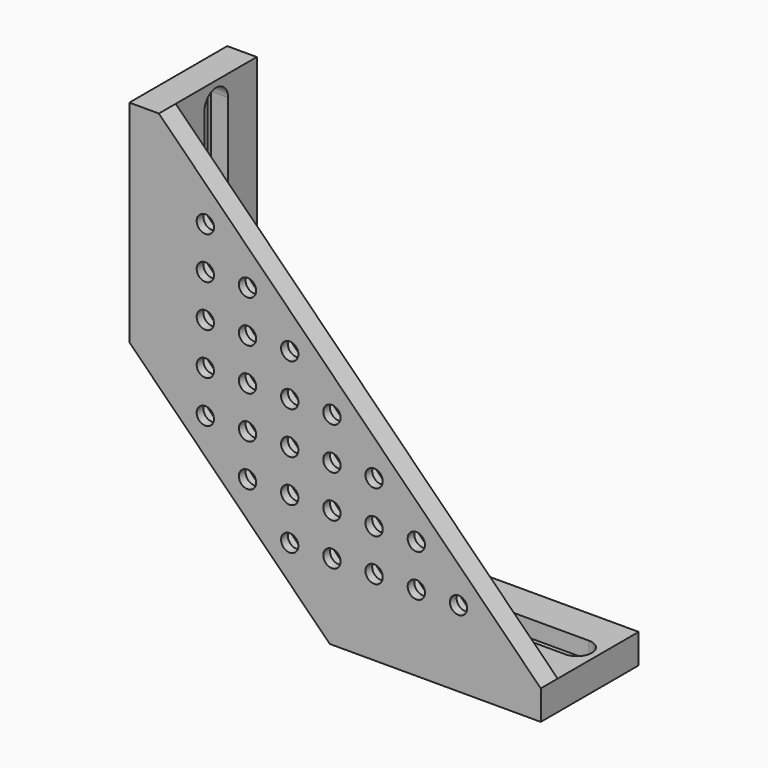
from build123d import *

# Parameters (mm, degrees)
F1_DEPTH  = 7
F2_DEPTH  = 3
F4_ANGLE  = 90
F8_ANGLE  = 180
F12_R     = 2.05
F13_DEPTH = 5
F14_DEPTH = 3


# Not quite as in the source:
# - a feature names something its author has since deleted; it is built from what else it names


with BuildPart() as f1:
    # F0 (on Top) → F1 (new body)
    with BuildSketch(Plane.XY):
        Polygon((29, 12), (-21, 12), (-21, -12), (0, -12), (29, -12), align=None)
        with BuildLine():
            ThreePointArc((-16, -11.5), (-19.5, -8), (-16, -4.5))
            Line((-16, -4.5), (0, -4.5))
            Line((0, -4.5), (24, -4.5))
            ThreePointArc((24, -4.5), (27.5, -8), (24, -11.5))
            Line((24, -11.5), (0, -11.5))
            Line((0, -11.5), (-16, -11.5))
        make_face(mode=Mode.SUBTRACT)
        with BuildLine():
            Line((24, -3.5), (-16, -3.5))
            ThreePointArc((-16, -3.5), (-19.5, 0), (-16, 3.5))
            Line((-16, 3.5), (24, 3.5))
            ThreePointArc((24, 3.5), (27.5, 0), (24, -3.5))
        make_face(mode=Mode.SUBTRACT)
        with BuildLine():
            Line((0, 4.5), (-16, 4.5))
            ThreePointArc((-16, 4.5), (-19.5, 8), (-16, 11.5))
            Line((-16, 11.5), (0, 11.5))
            Line((0, 11.5), (24, 11.5))
            ThreePointArc((24, 11.5), (27.5, 8), (24, 4.5))
            Line((24, 4.5), (0, 4.5))
        make_face(mode=Mode.SUBTRACT)
        with BuildLine():
            Line((0, -4.5), (-16, -4.5))
            ThreePointArc((-16, -4.5), (-19.5, -8), (-16, -11.5))
            Line((-16, -11.5), (0, -11.5))
            Line((0, -11.5), (24, -11.5))
            ThreePointArc((24, -11.5), (27.5, -8), (24, -4.5))
            Line((24, -4.5), (0, -4.5))
        make_face()
        with BuildLine():
            ThreePointArc((-16, -10.05), (-18.05, -8), (-16, -5.95))
            Line((-16, -5.95), (0, -5.95))
            Line((0, -5.95), (24, -5.95))
            ThreePointArc((24, -5.95), (26.05, -8), (24, -10.05))
            Line((24, -10.05), (0, -10.05))
            Line((0, -10.05), (-16, -10.05))
        make_face(mode=Mode.SUBTRACT)
        with BuildLine():
            ThreePointArc((-16, 11.5), (-19.5, 8), (-16, 4.5))
            Line((-16, 4.5), (0, 4.5))
            Line((0, 4.5), (24, 4.5))
            ThreePointArc((24, 4.5), (27.5, 8), (24, 11.5))
            Line((24, 11.5), (0, 11.5))
            Line((0, 11.5), (-16, 11.5))
        make_face()
        with BuildLine():
            Line((24, 5.95), (0, 5.95))
            Line((0, 5.95), (-16, 5.95))
            ThreePointArc((-16, 5.95), (-18.05, 8), (-16, 10.05))
            Line((-16, 10.05), (0, 10.05))
            Line((0, 10.05), (24, 10.05))
            ThreePointArc((24, 10.05), (26.05, 8), (24, 5.95))
        make_face(mode=Mode.SUBTRACT)
        with BuildLine():
            Line((0, -5.95), (-16, -5.95))
            ThreePointArc((-16, -5.95), (-18.05, -8), (-16, -10.05))
            Line((-16, -10.05), (0, -10.05))
            Line((0, -10.05), (24, -10.05))
            ThreePointArc((24, -10.05), (26.05, -8), (24, -5.95))
            Line((24, -5.95), (0, -5.95))
        make_face()
        with BuildLine():
            Line((-16, 5.95), (0, 5.95))
            Line((0, 5.95), (24, 5.95))
            ThreePointArc((24, 5.95), (26.05, 8), (24, 10.05))
            Line((24, 10.05), (0, 10.05))
            Line((0, 10.05), (-16, 10.05))
            ThreePointArc((-16, 10.05), (-18.05, 8), (-16, 5.95))
        make_face()
    extrude(amount=F1_DEPTH)

    # F0 (on Top) → F2 (join)
    with BuildSketch(Plane.XY):
        with BuildLine():
            ThreePointArc((-16, 3.5), (-19.5, 0), (-16, -3.5))
            Line((-16, -3.5), (24, -3.5))
            ThreePointArc((24, -3.5), (27.5, 0), (24, 3.5))
            Line((24, 3.5), (-16, 3.5))
        make_face()
        with BuildLine():
            Line((0, -2.45), (-16, -2.45))
            ThreePointArc((-16, -2.45), (-18.45, 0), (-16, 2.45))
            Line((-16, 2.45), (0, 2.45))
            Line((0, 2.45), (24, 2.45))
            ThreePointArc((24, 2.45), (26.45, 0), (24, -2.45))
            Line((24, -2.45), (0, -2.45))
        make_face(mode=Mode.SUBTRACT)
    extrude(amount=F2_DEPTH)


with BuildPart() as f4_1:
    # F4: copy of F1
    add(f1.part.rotate(Axis((-21, 0, 3.5), (0, -1, 0)), F4_ANGLE))


with BuildPart() as f4_1_1:
    # F8: moved
    add(f4_1.part.rotate(Axis((-21, 0, 28.5), (0, 0, 1)), F8_ANGLE))


with BuildPart() as f4_1_2:
    # F9: moved
    add(f4_1_1.part.moved(Location((0, 0, 44))))


with BuildPart() as f4_1_3:
    # F10: moved
    add(f4_1_2.part.moved(Location((-44, 0, 0))))


with BuildPart() as f1_1:
    add(f1.part)

    add(f4_1_3.part)  # F13 merges F4_1
    # F12 (on 3pt) → F13 (join)
    with BuildSketch(Plane.XZ.offset(12)):
        Polygon((-68.5, 47.5), (-21, 0), (29, 0), (29, 7), (-61.5, 97.5), (-68.5, 97.5), align=None)
        Polygon((-34.3563439923, 16.9720831325), (-33.3210678119, 20.8357864376), (-29.4573645067, 21.871062618), (-26.628937382, 19.0426354933), (-27.6642135624, 15.1789321881), (-31.5279168675, 14.1436560077), align=None, mode=Mode.SUBTRACT)
        Polygon((-24.3563439923, 16.9720831325), (-23.3210678119, 20.8357864376), (-19.4573645067, 21.871062618), (-16.628937382, 19.0426354933), (-17.6642135624, 15.1789321881), (-21.5279168675, 14.1436560077), align=None, mode=Mode.SUBTRACT)
        Polygon((-54.3563439923, 36.9720831325), (-53.3210678119, 40.8357864376), (-49.4573645067, 41.871062618), (-46.628937382, 39.0426354933), (-47.6642135624, 35.1789321881), (-51.5279168675, 34.1436560077), align=None, mode=Mode.SUBTRACT)
        Polygon((-54.3563439923, 46.9720831325), (-53.3210678119, 50.8357864376), (-49.4573645067, 51.871062618), (-46.628937382, 49.0426354933), (-47.6642135624, 45.1789321881), (-51.5279168675, 44.1436560077), align=None, mode=Mode.SUBTRACT)
        Polygon((-44.3563439923, 26.9720831325), (-43.3210678119, 30.8357864376), (-39.4573645067, 31.871062618), (-36.628937382, 29.0426354933), (-37.6642135624, 25.1789321881), (-41.5279168675, 24.1436560077), align=None, mode=Mode.SUBTRACT)
        Polygon((-34.3563439923, 26.9720831325), (-33.3210678119, 30.8357864376), (-29.4573645067, 31.871062618), (-26.628937382, 29.0426354933), (-27.6642135624, 25.1789321881), (-31.5279168675, 24.1436560077), align=None, mode=Mode.SUBTRACT)
        Polygon((-24.3563439923, 26.9720831325), (-23.3210678119, 30.8357864376), (-19.4573645067, 31.871062618), (-16.628937382, 29.0426354933), (-17.6642135624, 25.1789321881), (-21.5279168675, 24.1436560077), align=None, mode=Mode.SUBTRACT)
        Polygon((-44.3563439923, 36.9720831325), (-43.3210678119, 40.8357864376), (-39.4573645067, 41.871062618), (-36.628937382, 39.0426354933), (-37.6642135624, 35.1789321881), (-41.5279168675, 34.1436560077), align=None, mode=Mode.SUBTRACT)
        Polygon((-44.3563439923, 46.9720831325), (-43.3210678119, 50.8357864376), (-39.4573645067, 51.871062618), (-36.628937382, 49.0426354933), (-37.6642135624, 45.1789321881), (-41.5279168675, 44.1436560077), align=None, mode=Mode.SUBTRACT)
        Polygon((-34.3563439923, 36.9720831325), (-33.3210678119, 40.8357864376), (-29.4573645067, 41.871062618), (-26.628937382, 39.0426354933), (-27.6642135624, 35.1789321881), (-31.5279168675, 34.1436560077), align=None, mode=Mode.SUBTRACT)
        Polygon((-24.3563439923, 36.9720831325), (-23.3210678119, 40.8357864376), (-19.4573645067, 41.871062618), (-16.628937382, 39.0426354933), (-17.6642135624, 35.1789321881), (-21.5279168675, 34.1436560077), align=None, mode=Mode.SUBTRACT)
        Polygon((-34.3563439923, 46.9720831325), (-33.3210678119, 50.8357864376), (-29.4573645067, 51.871062618), (-26.628937382, 49.0426354933), (-27.6642135624, 45.1789321881), (-31.5279168675, 44.1436560077), align=None, mode=Mode.SUBTRACT)
        Polygon((-24.3563439923, 46.9720831325), (-23.3210678119, 50.8357864376), (-19.4573645067, 51.871062618), (-16.628937382, 49.0426354933), (-17.6642135624, 45.1789321881), (-21.5279168675, 44.1436560077), align=None, mode=Mode.SUBTRACT)
        Polygon((-14.3563439923, 16.9720831325), (-13.3210678119, 20.8357864376), (-9.4573645067, 21.871062618), (-6.628937382, 19.0426354933), (-7.6642135624, 15.1789321881), (-11.5279168675, 14.1436560077), align=None, mode=Mode.SUBTRACT)
        Polygon((-4.3563439923, 16.9720831325), (-3.3210678119, 20.8357864376), (0.5426354933, 21.871062618), (3.371062618, 19.0426354933), (2.3357864376, 15.1789321881), (-1.5279168675, 14.1436560077), align=None, mode=Mode.SUBTRACT)
        Polygon((8.4720831325, 14.1436560077), (5.6436560077, 16.9720831325), (6.6789321881, 20.8357864376), (10.5426354933, 21.871062618), (13.371062618, 19.0426354933), (12.3357864376, 15.1789321881), align=None, mode=Mode.SUBTRACT)
        Polygon((-14.3563439923, 26.9720831325), (-13.3210678119, 30.8357864376), (-9.4573645067, 31.871062618), (-6.628937382, 29.0426354933), (-7.6642135624, 25.1789321881), (-11.5279168675, 24.1436560077), align=None, mode=Mode.SUBTRACT)
        Polygon((-4.3563439923, 26.9720831325), (-3.3210678119, 30.8357864376), (0.5426354933, 31.871062618), (3.371062618, 29.0426354933), (2.3357864376, 25.1789321881), (-1.5279168675, 24.1436560077), align=None, mode=Mode.SUBTRACT)
        Polygon((-14.3563439923, 36.9720831325), (-13.3210678119, 40.8357864376), (-9.4573645067, 41.871062618), (-6.628937382, 39.0426354933), (-7.6642135624, 35.1789321881), (-11.5279168675, 34.1436560077), align=None, mode=Mode.SUBTRACT)
        Polygon((-54.3563439923, 56.9720831325), (-53.3210678119, 60.8357864376), (-49.4573645067, 61.871062618), (-46.628937382, 59.0426354933), (-47.6642135624, 55.1789321881), (-51.5279168675, 54.1436560077), align=None, mode=Mode.SUBTRACT)
        Polygon((-54.3563439923, 66.9720831325), (-53.3210678119, 70.8357864376), (-49.4573645067, 71.871062618), (-46.628937382, 69.0426354933), (-47.6642135624, 65.1789321881), (-51.5279168675, 64.1436560077), align=None, mode=Mode.SUBTRACT)
        Polygon((-44.3563439923, 56.9720831325), (-43.3210678119, 60.8357864376), (-39.4573645067, 61.871062618), (-36.628937382, 59.0426354933), (-37.6642135624, 55.1789321881), (-41.5279168675, 54.1436560077), align=None, mode=Mode.SUBTRACT)
        Polygon((-34.3563439923, 56.9720831325), (-33.3210678119, 60.8357864376), (-29.4573645067, 61.871062618), (-26.628937382, 59.0426354933), (-27.6642135624, 55.1789321881), (-31.5279168675, 54.1436560077), align=None, mode=Mode.SUBTRACT)
        Polygon((-41.5279168675, 64.1436560077), (-44.3563439923, 66.9720831325), (-43.3210678119, 70.8357864376), (-39.4573645067, 71.871062618), (-36.628937382, 69.0426354933), (-37.6642135624, 65.1789321881), align=None, mode=Mode.SUBTRACT)
        Polygon((-51.5279168675, 74.1436560077), (-54.3563439923, 76.9720831325), (-53.3210678119, 80.8357864376), (-49.4573645067, 81.871062618), (-46.628937382, 79.0426354933), (-47.6642135624, 75.1789321881), align=None, mode=Mode.SUBTRACT)
        Polygon((-19.4573645067, 51.871062618), (-23.3210678119, 50.8357864376), (-24.3563439923, 46.9720831325), (-21.5279168675, 44.1436560077), (-17.6642135624, 45.1789321881), (-16.628937382, 49.0426354933), align=None)
        with Locations((-20.4926406871, 48.0073593129)):
            Circle(F12_R, mode=Mode.SUBTRACT)
        Polygon((-29.4573645067, 61.871062618), (-33.3210678119, 60.8357864376), (-34.3563439923, 56.9720831325), (-31.5279168675, 54.1436560077), (-27.6642135624, 55.1789321881), (-26.628937382, 59.0426354933), align=None)
        with Locations((-30.4926406871, 58.0073593129)):
            Circle(F12_R, mode=Mode.SUBTRACT)
        Polygon((-29.4573645067, 51.871062618), (-33.3210678119, 50.8357864376), (-34.3563439923, 46.9720831325), (-31.5279168675, 44.1436560077), (-27.6642135624, 45.1789321881), (-26.628937382, 49.0426354933), align=None)
        with Locations((-30.4926406871, 48.0073593129)):
            Circle(F12_R, mode=Mode.SUBTRACT)
        Polygon((-29.4573645067, 41.871062618), (-33.3210678119, 40.8357864376), (-34.3563439923, 36.9720831325), (-31.5279168675, 34.1436560077), (-27.6642135624, 35.1789321881), (-26.628937382, 39.0426354933), align=None)
        with Locations((-30.4926406871, 38.0073593129)):
            Circle(F12_R, mode=Mode.SUBTRACT)
        Polygon((-19.4573645067, 41.871062618), (-23.3210678119, 40.8357864376), (-24.3563439923, 36.9720831325), (-21.5279168675, 34.1436560077), (-17.6642135624, 35.1789321881), (-16.628937382, 39.0426354933), align=None)
        with Locations((-20.4926406871, 38.0073593129)):
            Circle(F12_R, mode=Mode.SUBTRACT)
        Polygon((-9.4573645067, 41.871062618), (-13.3210678119, 40.8357864376), (-14.3563439923, 36.9720831325), (-11.5279168675, 34.1436560077), (-7.6642135624, 35.1789321881), (-6.628937382, 39.0426354933), align=None)
        with Locations((-10.4926406871, 38.0073593129)):
            Circle(F12_R, mode=Mode.SUBTRACT)
        Polygon((-43.3210678119, 70.8357864376), (-44.3563439923, 66.9720831325), (-41.5279168675, 64.1436560077), (-37.6642135624, 65.1789321881), (-36.628937382, 69.0426354933), (-39.4573645067, 71.871062618), align=None)
        with Locations((-40.4926406871, 68.0073593129)):
            Circle(F12_R, mode=Mode.SUBTRACT)
        Polygon((-39.4573645067, 61.871062618), (-43.3210678119, 60.8357864376), (-44.3563439923, 56.9720831325), (-41.5279168675, 54.1436560077), (-37.6642135624, 55.1789321881), (-36.628937382, 59.0426354933), align=None)
        with Locations((-40.4926406871, 58.0073593129)):
            Circle(F12_R, mode=Mode.SUBTRACT)
        Polygon((-39.4573645067, 51.871062618), (-43.3210678119, 50.8357864376), (-44.3563439923, 46.9720831325), (-41.5279168675, 44.1436560077), (-37.6642135624, 45.1789321881), (-36.628937382, 49.0426354933), align=None)
        with Locations((-40.4926406871, 48.0073593129)):
            Circle(F12_R, mode=Mode.SUBTRACT)
        Polygon((-39.4573645067, 41.871062618), (-43.3210678119, 40.8357864376), (-44.3563439923, 36.9720831325), (-41.5279168675, 34.1436560077), (-37.6642135624, 35.1789321881), (-36.628937382, 39.0426354933), align=None)
        with Locations((-40.4926406871, 38.0073593129)):
            Circle(F12_R, mode=Mode.SUBTRACT)
        Polygon((-39.4573645067, 31.871062618), (-43.3210678119, 30.8357864376), (-44.3563439923, 26.9720831325), (-41.5279168675, 24.1436560077), (-37.6642135624, 25.1789321881), (-36.628937382, 29.0426354933), align=None)
        with Locations((-40.4926406871, 28.0073593129)):
            Circle(F12_R, mode=Mode.SUBTRACT)
        Polygon((-29.4573645067, 31.871062618), (-33.3210678119, 30.8357864376), (-34.3563439923, 26.9720831325), (-31.5279168675, 24.1436560077), (-27.6642135624, 25.1789321881), (-26.628937382, 29.0426354933), align=None)
        with Locations((-30.4926406871, 28.0073593129)):
            Circle(F12_R, mode=Mode.SUBTRACT)
        Polygon((-19.4573645067, 31.871062618), (-23.3210678119, 30.8357864376), (-24.3563439923, 26.9720831325), (-21.5279168675, 24.1436560077), (-17.6642135624, 25.1789321881), (-16.628937382, 29.0426354933), align=None)
        with Locations((-20.4926406871, 28.0073593129)):
            Circle(F12_R, mode=Mode.SUBTRACT)
        Polygon((-9.4573645067, 31.871062618), (-13.3210678119, 30.8357864376), (-14.3563439923, 26.9720831325), (-11.5279168675, 24.1436560077), (-7.6642135624, 25.1789321881), (-6.628937382, 29.0426354933), align=None)
        with Locations((-10.4926406871, 28.0073593129)):
            Circle(F12_R, mode=Mode.SUBTRACT)
        Polygon((0.5426354933, 31.871062618), (-3.3210678119, 30.8357864376), (-4.3563439923, 26.9720831325), (-1.5279168675, 24.1436560077), (2.3357864376, 25.1789321881), (3.371062618, 29.0426354933), align=None)
        with Locations((-0.4926406871, 28.0073593129)):
            Circle(F12_R, mode=Mode.SUBTRACT)
        Polygon((-49.4573645067, 61.871062618), (-53.3210678119, 60.8357864376), (-54.3563439923, 56.9720831325), (-51.5279168675, 54.1436560077), (-47.6642135624, 55.1789321881), (-46.628937382, 59.0426354933), align=None)
        with Locations((-50.4926406871, 58.0073593129)):
            Circle(F12_R, mode=Mode.SUBTRACT)
        Polygon((-49.4573645067, 71.871062618), (-53.3210678119, 70.8357864376), (-54.3563439923, 66.9720831325), (-51.5279168675, 64.1436560077), (-47.6642135624, 65.1789321881), (-46.628937382, 69.0426354933), align=None)
        with Locations((-50.4926406871, 68.0073593129)):
            Circle(F12_R, mode=Mode.SUBTRACT)
        Polygon((-53.3210678119, 80.8357864376), (-54.3563439923, 76.9720831325), (-51.5279168675, 74.1436560077), (-47.6642135624, 75.1789321881), (-46.628937382, 79.0426354933), (-49.4573645067, 81.871062618), align=None)
        with Locations((-50.4926406871, 78.0073593129)):
            Circle(F12_R, mode=Mode.SUBTRACT)
        Polygon((-49.4573645067, 51.871062618), (-53.3210678119, 50.8357864376), (-54.3563439923, 46.9720831325), (-51.5279168675, 44.1436560077), (-47.6642135624, 45.1789321881), (-46.628937382, 49.0426354933), align=None)
        with Locations((-50.4926406871, 48.0073593129)):
            Circle(F12_R, mode=Mode.SUBTRACT)
        Polygon((-49.4573645067, 41.871062618), (-53.3210678119, 40.8357864376), (-54.3563439923, 36.9720831325), (-51.5279168675, 34.1436560077), (-47.6642135624, 35.1789321881), (-46.628937382, 39.0426354933), align=None)
        with Locations((-50.4926406871, 38.0073593129)):
            Circle(F12_R, mode=Mode.SUBTRACT)
        Polygon((-29.4573645067, 21.871062618), (-33.3210678119, 20.8357864376), (-34.3563439923, 16.9720831325), (-31.5279168675, 14.1436560077), (-27.6642135624, 15.1789321881), (-26.628937382, 19.0426354933), align=None)
        with Locations((-30.4926406871, 18.0073593129)):
            Circle(F12_R, mode=Mode.SUBTRACT)
        Polygon((-19.4573645067, 21.871062618), (-23.3210678119, 20.8357864376), (-24.3563439923, 16.9720831325), (-21.5279168675, 14.1436560077), (-17.6642135624, 15.1789321881), (-16.628937382, 19.0426354933), align=None)
        with Locations((-20.4926406871, 18.0073593129)):
            Circle(F12_R, mode=Mode.SUBTRACT)
        Polygon((-9.4573645067, 21.871062618), (-13.3210678119, 20.8357864376), (-14.3563439923, 16.9720831325), (-11.5279168675, 14.1436560077), (-7.6642135624, 15.1789321881), (-6.628937382, 19.0426354933), align=None)
        with Locations((-10.4926406871, 18.0073593129)):
            Circle(F12_R, mode=Mode.SUBTRACT)
        Polygon((0.5426354933, 21.871062618), (-3.3210678119, 20.8357864376), (-4.3563439923, 16.9720831325), (-1.5279168675, 14.1436560077), (2.3357864376, 15.1789321881), (3.371062618, 19.0426354933), align=None)
        with Locations((-0.4926406871, 18.0073593129)):
            Circle(F12_R, mode=Mode.SUBTRACT)
        Polygon((6.6789321881, 20.8357864376), (5.6436560077, 16.9720831325), (8.4720831325, 14.1436560077), (12.3357864376, 15.1789321881), (13.371062618, 19.0426354933), (10.5426354933, 21.871062618), align=None)
        with Locations((9.5073593129, 18.0073593129)):
            Circle(F12_R, mode=Mode.SUBTRACT)
    extrude(amount=F13_DEPTH)

    # F12 (on 3pt) → F14 (cut)
    with BuildSketch(Plane.XZ.offset(12)):
        Polygon((-19.4573645067, 51.871062618), (-23.3210678119, 50.8357864376), (-24.3563439923, 46.9720831325), (-21.5279168675, 44.1436560077), (-17.6642135624, 45.1789321881), (-16.628937382, 49.0426354933), align=None)
        with Locations((-20.4926406871, 48.0073593129)):
            Circle(F12_R, mode=Mode.SUBTRACT)
        Polygon((-9.4573645067, 41.871062618), (-13.3210678119, 40.8357864376), (-14.3563439923, 36.9720831325), (-11.5279168675, 34.1436560077), (-7.6642135624, 35.1789321881), (-6.628937382, 39.0426354933), align=None)
        with Locations((-10.4926406871, 38.0073593129)):
            Circle(F12_R, mode=Mode.SUBTRACT)
        Polygon((-19.4573645067, 41.871062618), (-23.3210678119, 40.8357864376), (-24.3563439923, 36.9720831325), (-21.5279168675, 34.1436560077), (-17.6642135624, 35.1789321881), (-16.628937382, 39.0426354933), align=None)
        with Locations((-20.4926406871, 38.0073593129)):
            Circle(F12_R, mode=Mode.SUBTRACT)
        Polygon((-29.4573645067, 41.871062618), (-33.3210678119, 40.8357864376), (-34.3563439923, 36.9720831325), (-31.5279168675, 34.1436560077), (-27.6642135624, 35.1789321881), (-26.628937382, 39.0426354933), align=None)
        with Locations((-30.4926406871, 38.0073593129)):
            Circle(F12_R, mode=Mode.SUBTRACT)
        Polygon((-29.4573645067, 51.871062618), (-33.3210678119, 50.8357864376), (-34.3563439923, 46.9720831325), (-31.5279168675, 44.1436560077), (-27.6642135624, 45.1789321881), (-26.628937382, 49.0426354933), align=None)
        with Locations((-30.4926406871, 48.0073593129)):
            Circle(F12_R, mode=Mode.SUBTRACT)
        Polygon((-29.4573645067, 61.871062618), (-33.3210678119, 60.8357864376), (-34.3563439923, 56.9720831325), (-31.5279168675, 54.1436560077), (-27.6642135624, 55.1789321881), (-26.628937382, 59.0426354933), align=None)
        with Locations((-30.4926406871, 58.0073593129)):
            Circle(F12_R, mode=Mode.SUBTRACT)
        Polygon((0.5426354933, 31.871062618), (-3.3210678119, 30.8357864376), (-4.3563439923, 26.9720831325), (-1.5279168675, 24.1436560077), (2.3357864376, 25.1789321881), (3.371062618, 29.0426354933), align=None)
        with Locations((-0.4926406871, 28.0073593129)):
            Circle(F12_R, mode=Mode.SUBTRACT)
        Polygon((-9.4573645067, 31.871062618), (-13.3210678119, 30.8357864376), (-14.3563439923, 26.9720831325), (-11.5279168675, 24.1436560077), (-7.6642135624, 25.1789321881), (-6.628937382, 29.0426354933), align=None)
        with Locations((-10.4926406871, 28.0073593129)):
            Circle(F12_R, mode=Mode.SUBTRACT)
        Polygon((-19.4573645067, 31.871062618), (-23.3210678119, 30.8357864376), (-24.3563439923, 26.9720831325), (-21.5279168675, 24.1436560077), (-17.6642135624, 25.1789321881), (-16.628937382, 29.0426354933), align=None)
        with Locations((-20.4926406871, 28.0073593129)):
            Circle(F12_R, mode=Mode.SUBTRACT)
        Polygon((-29.4573645067, 31.871062618), (-33.3210678119, 30.8357864376), (-34.3563439923, 26.9720831325), (-31.5279168675, 24.1436560077), (-27.6642135624, 25.1789321881), (-26.628937382, 29.0426354933), align=None)
        with Locations((-30.4926406871, 28.0073593129)):
            Circle(F12_R, mode=Mode.SUBTRACT)
        Polygon((-39.4573645067, 31.871062618), (-43.3210678119, 30.8357864376), (-44.3563439923, 26.9720831325), (-41.5279168675, 24.1436560077), (-37.6642135624, 25.1789321881), (-36.628937382, 29.0426354933), align=None)
        with Locations((-40.4926406871, 28.0073593129)):
            Circle(F12_R, mode=Mode.SUBTRACT)
        Polygon((-39.4573645067, 41.871062618), (-43.3210678119, 40.8357864376), (-44.3563439923, 36.9720831325), (-41.5279168675, 34.1436560077), (-37.6642135624, 35.1789321881), (-36.628937382, 39.0426354933), align=None)
        with Locations((-40.4926406871, 38.0073593129)):
            Circle(F12_R, mode=Mode.SUBTRACT)
        Polygon((-39.4573645067, 51.871062618), (-43.3210678119, 50.8357864376), (-44.3563439923, 46.9720831325), (-41.5279168675, 44.1436560077), (-37.6642135624, 45.1789321881), (-36.628937382, 49.0426354933), align=None)
        with Locations((-40.4926406871, 48.0073593129)):
            Circle(F12_R, mode=Mode.SUBTRACT)
        Polygon((-39.4573645067, 61.871062618), (-43.3210678119, 60.8357864376), (-44.3563439923, 56.9720831325), (-41.5279168675, 54.1436560077), (-37.6642135624, 55.1789321881), (-36.628937382, 59.0426354933), align=None)
        with Locations((-40.4926406871, 58.0073593129)):
            Circle(F12_R, mode=Mode.SUBTRACT)
        Polygon((-43.3210678119, 70.8357864376), (-44.3563439923, 66.9720831325), (-41.5279168675, 64.1436560077), (-37.6642135624, 65.1789321881), (-36.628937382, 69.0426354933), (-39.4573645067, 71.871062618), align=None)
        with Locations((-40.4926406871, 68.0073593129)):
            Circle(F12_R, mode=Mode.SUBTRACT)
        Polygon((-53.3210678119, 80.8357864376), (-54.3563439923, 76.9720831325), (-51.5279168675, 74.1436560077), (-47.6642135624, 75.1789321881), (-46.628937382, 79.0426354933), (-49.4573645067, 81.871062618), align=None)
        with Locations((-50.4926406871, 78.0073593129)):
            Circle(F12_R, mode=Mode.SUBTRACT)
        Polygon((-49.4573645067, 71.871062618), (-53.3210678119, 70.8357864376), (-54.3563439923, 66.9720831325), (-51.5279168675, 64.1436560077), (-47.6642135624, 65.1789321881), (-46.628937382, 69.0426354933), align=None)
        with Locations((-50.4926406871, 68.0073593129)):
            Circle(F12_R, mode=Mode.SUBTRACT)
        Polygon((-49.4573645067, 61.871062618), (-53.3210678119, 60.8357864376), (-54.3563439923, 56.9720831325), (-51.5279168675, 54.1436560077), (-47.6642135624, 55.1789321881), (-46.628937382, 59.0426354933), align=None)
        with Locations((-50.4926406871, 58.0073593129)):
            Circle(F12_R, mode=Mode.SUBTRACT)
        Polygon((-49.4573645067, 51.871062618), (-53.3210678119, 50.8357864376), (-54.3563439923, 46.9720831325), (-51.5279168675, 44.1436560077), (-47.6642135624, 45.1789321881), (-46.628937382, 49.0426354933), align=None)
        with Locations((-50.4926406871, 48.0073593129)):
            Circle(F12_R, mode=Mode.SUBTRACT)
        Polygon((-49.4573645067, 41.871062618), (-53.3210678119, 40.8357864376), (-54.3563439923, 36.9720831325), (-51.5279168675, 34.1436560077), (-47.6642135624, 35.1789321881), (-46.628937382, 39.0426354933), align=None)
        with Locations((-50.4926406871, 38.0073593129)):
            Circle(F12_R, mode=Mode.SUBTRACT)
        Polygon((-29.4573645067, 21.871062618), (-33.3210678119, 20.8357864376), (-34.3563439923, 16.9720831325), (-31.5279168675, 14.1436560077), (-27.6642135624, 15.1789321881), (-26.628937382, 19.0426354933), align=None)
        with Locations((-30.4926406871, 18.0073593129)):
            Circle(F12_R, mode=Mode.SUBTRACT)
        Polygon((-19.4573645067, 21.871062618), (-23.3210678119, 20.8357864376), (-24.3563439923, 16.9720831325), (-21.5279168675, 14.1436560077), (-17.6642135624, 15.1789321881), (-16.628937382, 19.0426354933), align=None)
        with Locations((-20.4926406871, 18.0073593129)):
            Circle(F12_R, mode=Mode.SUBTRACT)
        Polygon((-9.4573645067, 21.871062618), (-13.3210678119, 20.8357864376), (-14.3563439923, 16.9720831325), (-11.5279168675, 14.1436560077), (-7.6642135624, 15.1789321881), (-6.628937382, 19.0426354933), align=None)
        with Locations((-10.4926406871, 18.0073593129)):
            Circle(F12_R, mode=Mode.SUBTRACT)
        Polygon((0.5426354933, 21.871062618), (-3.3210678119, 20.8357864376), (-4.3563439923, 16.9720831325), (-1.5279168675, 14.1436560077), (2.3357864376, 15.1789321881), (3.371062618, 19.0426354933), align=None)
        with Locations((-0.4926406871, 18.0073593129)):
            Circle(F12_R, mode=Mode.SUBTRACT)
        Polygon((6.6789321881, 20.8357864376), (5.6436560077, 16.9720831325), (8.4720831325, 14.1436560077), (12.3357864376, 15.1789321881), (13.371062618, 19.0426354933), (10.5426354933, 21.871062618), align=None)
        with Locations((9.5073593129, 18.0073593129)):
            Circle(F12_R, mode=Mode.SUBTRACT)
    extrude(amount=F14_DEPTH, mode=Mode.SUBTRACT)


solid = f1_1.part
